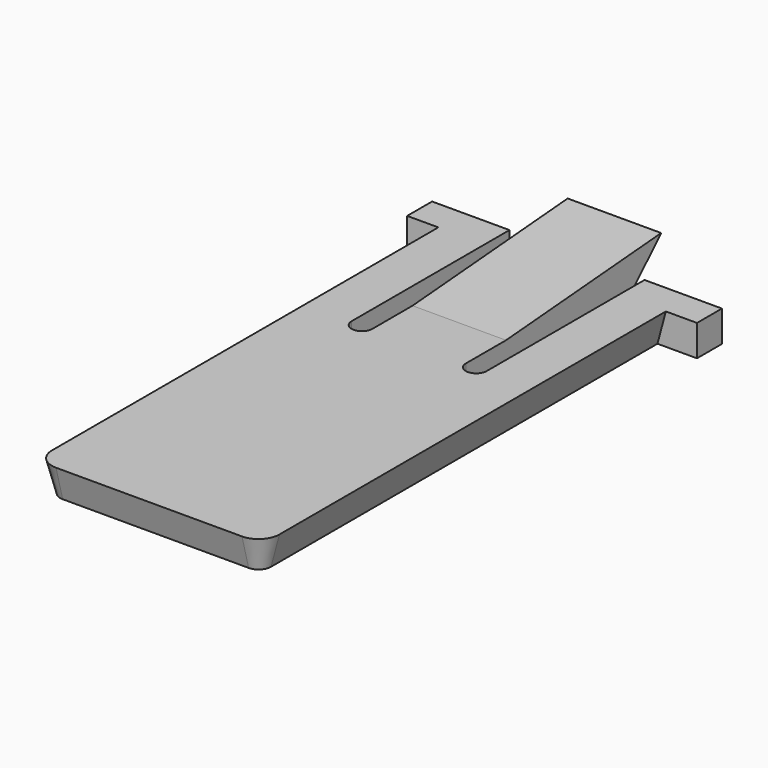
from build123d import *

# Parameters (mm, degrees)
F0_W     = 3
F0_H     = 3
F1_DEPTH = 3
F3_DEPTH = 4.5
F4_SIZE2 = 0.803838
F4_SIZE  = 2.99999


# Not quite as in the source:
# - a fillet or chamfer is up to 0.001 mm smaller than in the source, because OpenCascade refuses the exact size


with BuildPart() as f1:
    # F0 (on Top) → F1 (new body)
    with BuildSketch(Plane.XY):
        with BuildLine():
            Line((-6.5, 25.75), (-10.95, 25.75))
            Line((-10.95, 25.75), (-10.95, 22.75))
            Line((-10.95, 22.75), (-10.95, -23.75))
            ThreePointArc((-10.95, -23.75), (-10.3642135624, -25.1642135624), (-8.95, -25.75))
            Line((-8.95, -25.75), (8.95, -25.75))
            ThreePointArc((8.95, -25.75), (10.3642135624, -25.1642135624), (10.95, -23.75))
            Line((10.95, -23.75), (10.95, 22.75))
            Line((10.95, 22.75), (10.95, 25.75))
            Line((10.95, 25.75), (6.5, 25.75))
            Line((6.5, 25.75), (6.5, 6.75))
            ThreePointArc((6.5, 6.75), (6.2071067812, 6.0428932188), (5.5, 5.75))
            ThreePointArc((5.5, 5.75), (4.7928932188, 6.0428932188), (4.5, 6.75))
            Line((4.5, 6.75), (4.5, 25.75))
            Line((4.5, 25.75), (-4.5, 25.75))
            Line((-4.5, 25.75), (-4.5, 6.75))
            ThreePointArc((-4.5, 6.75), (-4.7928932188, 6.0428932188), (-5.5, 5.75))
            ThreePointArc((-5.5, 5.75), (-6.2071067812, 6.0428932188), (-6.5, 6.75))
            Line((-6.5, 6.75), (-6.5, 25.75))
        make_face()
        with Locations((-12.45, 24.25)):
            Rectangle(F0_W, F0_H)
        with Locations((12.45, 24.25)):
            Rectangle(F0_W, F0_H)
    extrude(amount=F1_DEPTH)

    # F2 (on Right) → F3 (join, symmetric)
    with BuildSketch(Plane.YZ):
        Polygon((-25.75, 0), (25.75, 0), (30.25, 4.5), align=None)
    extrude(amount=F3_DEPTH, both=True)

    # F4 (size 3 and 0.8038475773 in the source; OpenCascade refuses exactly that, so slightly less here)
    f4_edges = [f1.edges().sort_by_distance(p)[0] for p in [
        (0, -25.75, 0),
    ]]
    f4_side = f1.faces().sort_by_distance((0, -25.75, 1.5))[0]
    chamfer(f4_edges, length=F4_SIZE, length2=F4_SIZE2, reference=f4_side)


solid = f1.part
